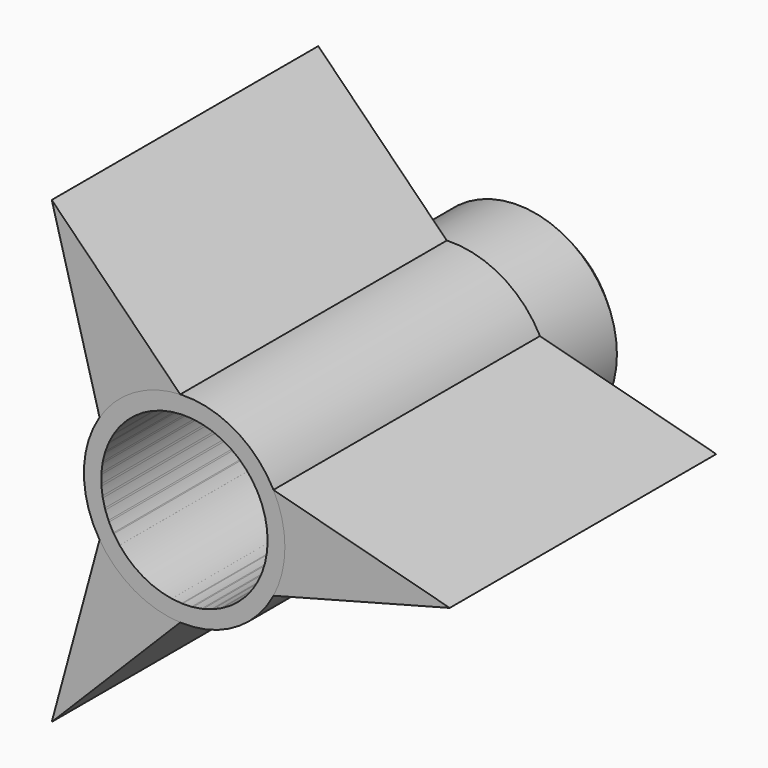
from build123d import *

# Parameters (mm, degrees)
F1_DEPTH = 25.4
F2_R     = 7.6630831302
F3_DEPTH = 25.4
F4_R     = 7.5760558817
F4_R_2   = 6.35
F5_DEPTH = 8.89
F7_R     = 6.3438436569
F8_DEPTH = 32.9770558817


# Not quite as in the source:
# - a fillet or chamfer that OpenCascade refuses, or shapes differently, is made with other operations: its cross-section is extruded or revolved along the edge and cut away or added


with BuildPart() as f1:
    # F0 (on Front) → F1 (new body)
    with BuildSketch(Plane.XZ):
        Polygon((-6.35, 3.6661742094), (-3.1749998817, 5.4992613823), (0, 7.3323484187), (-10.1139404636, 17.5178587477), align=None)
        with BuildLine():
            ThreePointArc((-6.35, 0), (-5.4992612799, 3.1750000591), (-3.1749998817, 5.4992613823))
            Line((-3.1749998817, 5.4992613823), (-6.35, 3.6661742094))
            Line((-6.35, 3.6661742094), (-6.35, 0))
        make_face()
        with BuildLine():
            ThreePointArc((-3.1749998817, 5.4992613823), (8.7e-08, 6.35), (3.1750000324, 5.4992612953))
            Line((3.1750000324, 5.4992612953), (0, 7.3323484187))
            Line((0, 7.3323484187), (-3.1749998817, 5.4992613823))
        make_face()
    extrude(amount=F1_DEPTH)


with BuildPart() as f1b:
    # F0 (on Front) → F1, piece 2 (new body)
    with BuildSketch(Plane.XZ):
        Polygon((6.35, 3.6661742094), (6.35, 0), (6.35, -3.6661742094), (20.2278809273, 0), align=None)
        with BuildLine():
            ThreePointArc((3.1750000324, 5.4992612953), (5.4992613234, 3.1749999838), (6.35, 0))
            Line((6.35, 0), (6.35, 3.6661742094))
            Line((6.35, 3.6661742094), (3.1750000324, 5.4992612953))
        make_face()
        with BuildLine():
            Line((6.35, -3.6661742094), (6.35, 0))
            ThreePointArc((6.35, 0), (5.4992612955, -3.175000032), (3.174999936, -5.499261351))
            Line((3.174999936, -5.499261351), (6.35, -3.6661742094))
        make_face()
    extrude(amount=F1_DEPTH)


with BuildPart() as f1c:
    # F0 (on Front) → F1, piece 3 (new body)
    with BuildSketch(Plane.XZ):
        Polygon((0, -7.3323484187), (-3.1749999956, -5.4992613166), (-6.35, -3.6661742094), (-10.1139404636, -17.5178587477), align=None)
        with BuildLine():
            Line((-6.35, -3.6661742094), (-3.1749999956, -5.4992613166))
            ThreePointArc((-3.1749999956, -5.4992613166), (-5.4992613128, -3.1750000022), (-6.35, 0))
            Line((-6.35, 0), (-6.35, -3.6661742094))
        make_face()
        with BuildLine():
            Line((0, -7.3323484187), (3.174999936, -5.499261351))
            ThreePointArc((3.174999936, -5.499261351), (-3.44e-08, -6.35), (-3.1749999956, -5.4992613166))
            Line((-3.1749999956, -5.4992613166), (0, -7.3323484187))
        make_face()
    extrude(amount=F1_DEPTH)


with BuildPart() as f3:
    # F2 (on Front) → F3 (new body)
    with BuildSketch(Plane.XZ):
        Circle(F2_R)
    extrude(amount=F3_DEPTH)

    # F7 (on face) → F8 (cut, through all)
    with BuildSketch(Plane.XZ.offset(25.4)):
        Circle(F7_R)
    extrude(amount=-F8_DEPTH, mode=Mode.SUBTRACT)


with BuildPart() as f5:
    # F4 (on Front) → F5 (new body)
    with BuildSketch(Plane.XZ):
        Circle(F4_R)
        Circle(F4_R_2, mode=Mode.SUBTRACT)
    extrude(amount=-F5_DEPTH)

    # F6: chamfer of 2.54 on 1 edges, made by hand

    # F6_s1 → F6_t2 (revolve, cut)
    with BuildSketch(Plane.XY):
        Polygon((7.5760558817, 6.35), (5.0360558817, 8.89), (7.5760558817, 8.89), align=None)
    revolve(axis=Axis((0, 8.89, 0), (0, -1, 0)), mode=Mode.SUBTRACT)


solid = Compound([f1.part, f1b.part, f1c.part, f3.part, f5.part])
